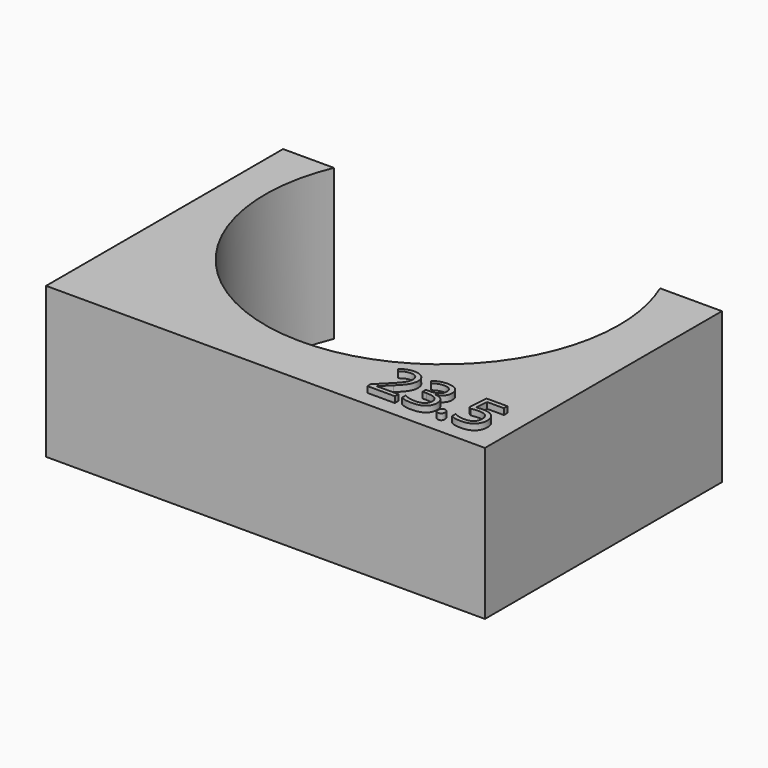
from build123d import *

# Parameters (mm, degrees)
F1_DEPTH     = 10
F4_TEXT_SIZE = 3.8808392775
F5_DEPTH     = 0.4


# Not quite as in the source:
# - Text() gives the source's letters only with a copy of the font that has no kerning and outlines rounded to 1/6400 em; it was checked with that copy


with BuildPart() as f1:
    # F0 (on Top) → F1 (new body)
    with BuildSketch(Plane.XY):
        with BuildLine():
            ThreePointArc((10.8313808286, 4.5545240527), (11.5180559283, 2.3231202363), (11.75, 0))
            ThreePointArc((11.75, 0), (-2.3231202363, -11.5180559283), (-10.8313808286, 4.5545240527))
            Line((-10.8313808286, 4.5545240527), (-14.210113143, 4.5545240527))
            Line((-14.210113143, 4.5545240527), (-14.210113143, -15.1210187458))
            Line((-14.210113143, -15.1210187458), (14.9388403982, -15.1210187458))
            Line((14.9388403982, -15.1210187458), (14.9388403982, 4.5545240527))
            Line((14.9388403982, 4.5545240527), (10.8313808286, 4.5545240527))
        make_face()
    extrude(amount=F1_DEPTH)


with BuildPart() as f2_1:
    # F2: copy of F1
    add(f1.part)


with BuildPart() as f1_1:
    add(f1.part)

    # F4 (on face) → F5 (join)
    with BuildSketch(Plane.XY.offset(10)):
        with Locations((6.1272741295, -14.1032282263)):
            Text('23.5', F4_TEXT_SIZE, font='Open Sans', text_align=(TextAlign.LEFT, TextAlign.BOTTOM))
    extrude(amount=F5_DEPTH)


solid = f1_1.part
